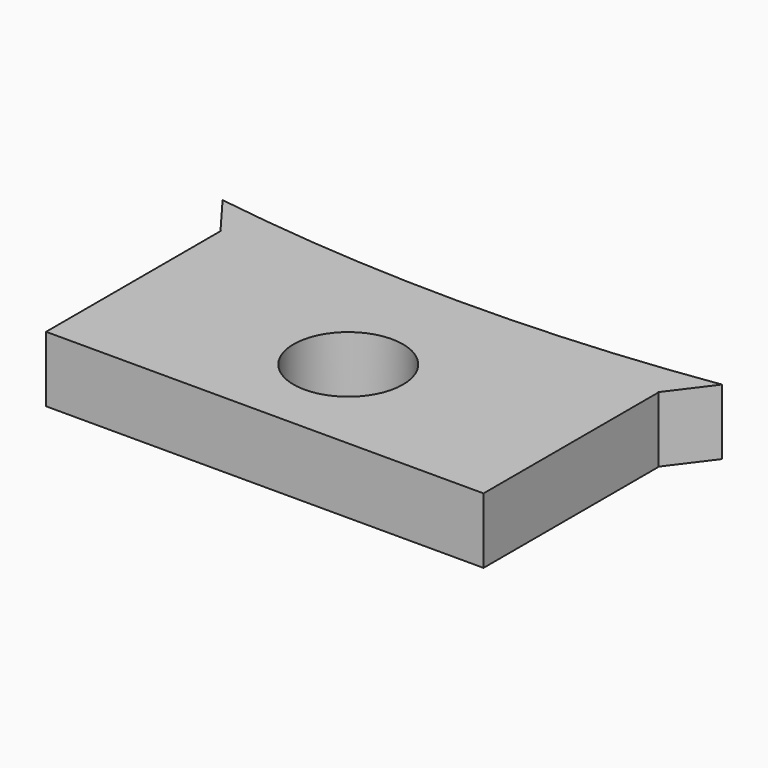
from build123d import *

# Parameters (mm, degrees)
F0_R     = 2.5
F1_DEPTH = 3


# Not quite as in the source:
# - a feature names something its author has since deleted; it is built from what else it names


with BuildPart() as f1:
    # F0 (on Top) → F1 (new body)
    with BuildSketch(Plane.XY):
        with BuildLine():
            Line((-14.8844467476, 9.0084131807), (-14.8591619832, 9.0084131807))
            Line((-14.8591619832, 9.0084131807), (5.1155532524, 9.0084131807))
            Line((5.1155532524, 9.0084131807), (6.5302648152, 10.8946952644))
            ThreePointArc((6.5302648152, 10.8946952644), (-4.8844467476, 10.0579512552), (-16.2991583104, 10.8946952644))
            Line((-16.2991583104, 10.8946952644), (-14.8844467476, 9.0084131807))
        make_face()
        Polygon((5.1155532524, 9.0084131807), (-14.8591619832, 9.0084131807), (-14.8591619832, -0.9915868193), (5.1408380168, -0.9915868193), (5.1408380168, 9.0084131807), align=None)
        with Locations((-4.8591619832, 3.7784131807)):
            Circle(F0_R, mode=Mode.SUBTRACT)
    extrude(amount=F1_DEPTH)


solid = f1.part
